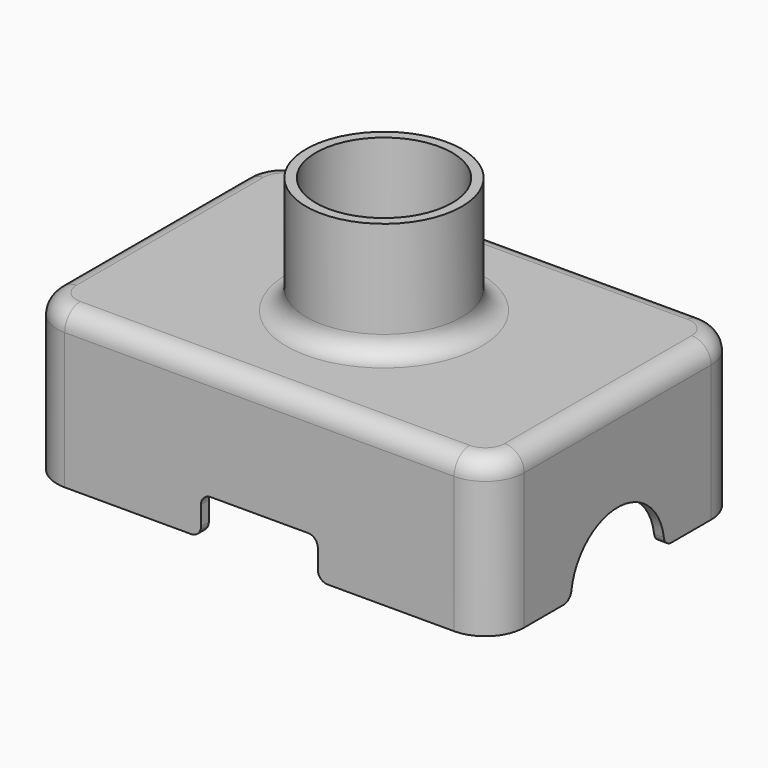
from build123d import *

# Parameters (mm, degrees)
F0_W         = 152.4
F0_H         = 101.6
F1_DEPTH     = 50.8
F2_R         = 25.4
F3_DEPTH     = 38.1
F4_R         = 12.7
F5_R         = 6.35
F6_T         = -3.175
F8_DEPTH     = 3.175
F9_W         = 38.1
F9_H         = 25.4
F10_DEPTH    = 3.175
F11_T1_DEPTH = 3.175
F11_T3_DEPTH = 17.9102262806
F11_T5_DEPTH = 19.05


# Not quite as in the source:
# - a fillet or chamfer that OpenCascade refuses, or shapes differently, is made with other operations: its cross-section is extruded or revolved along the edge and cut away or added


with BuildPart() as f1:
    # F0 (on Top) → F1 (new body)
    with BuildSketch(Plane.XY):
        Rectangle(F0_W, F0_H)
    extrude(amount=F1_DEPTH)

    # F2 (on face) → F3 (join)
    with BuildSketch(Plane.XY.offset(50.8)):
        Circle(F2_R)
    extrude(amount=F3_DEPTH)

    # F4
    f4_edges = [f1.edges().sort_by_distance(p)[0] for p in [
        (-76.2, -50.8, 25.4),
        (76.2, -50.8, 25.4),
        (76.2, 50.8, 25.4),
        (-76.2, 50.8, 25.4),
    ]]
    fillet(f4_edges, radius=F4_R)

    # F5
    f5_edges = [f1.edges().sort_by_distance(p)[0] for p in [
        (-25.4, 0, 50.8),
        (76.2, 0, 50.8),
        (72.480256, -47.080256, 50.8),
        (72.480256, 47.080256, 50.8),
        (0, -50.8, 50.8),
        (0, 50.8, 50.8),
        (-72.480256, -47.080256, 50.8),
        (-72.480256, 47.080256, 50.8),
        (-76.2, 0, 50.8),
    ]]
    fillet(f5_edges, radius=F5_R)

    # F6
    f6_openings = [f1.faces().sort_by_distance(p)[0] for p in [
        (0, 0, 0),
        (0, 0, 88.9),
    ]]
    offset(amount=F6_T, openings=f6_openings)

    # F7 (on face) → F8 (cut, through all)
    with BuildSketch(Plane.YZ.offset(76.2)):
        with BuildLine():
            Line((-19.05, 0), (19.05, 0))
            ThreePointArc((19.05, 0), (0, 19.05), (-19.05, 0))
        make_face()
    extrude(amount=-F8_DEPTH, mode=Mode.SUBTRACT)

    # F9 (on face) → F10 (cut, through all)
    with BuildSketch(Plane.XZ.offset(50.8)):
        Rectangle(F9_W, F9_H)
    extrude(amount=-F10_DEPTH, mode=Mode.SUBTRACT)

    # F11: fillet of radius 3.175 on 8 edges, made by hand

    # F11_s2 → F11_t1 (join)
    with BuildSketch(Plane.XZ.offset(47.625)):
        with BuildLine():
            ThreePointArc((-19.05, 9.525), (-18.1200640303, 11.7700640303), (-15.875, 12.7))
            Line((-15.875, 12.7), (-19.05, 12.7))
            Line((-19.05, 12.7), (-19.05, 9.525))
        make_face()
        with BuildLine():
            ThreePointArc((19.05, 9.525), (18.1200640303, 11.7700640303), (15.875, 12.7))
            Line((15.875, 12.7), (19.05, 12.7))
            Line((19.05, 12.7), (19.05, 9.525))
        make_face()
    extrude(amount=F11_T1_DEPTH)

    # F11_s4 → F11_t3 (cut)
    with BuildSketch(Plane.YZ.offset(65.6573868597)):
        with BuildLine():
            ThreePointArc((-21.9970452561, 0), (-19.9185198516, 0.7749255964), (-18.8546102195, 2.7214285714))
            ThreePointArc((-18.8546102195, 2.7214285714), (-19.0010897672, 1.3642168665), (-19.05, 0))
            Line((-19.05, 0), (-21.9970452561, 0))
        make_face()
        with BuildLine():
            ThreePointArc((18.8546102195, 2.7214285714), (19.9185198516, 0.7749255964), (21.9970452561, 0))
            Line((21.9970452561, 0), (19.05, 0))
            ThreePointArc((19.05, 0), (19.0010897672, 1.3642168665), (18.8546102195, 2.7214285714))
        make_face()
    extrude(amount=F11_T3_DEPTH, mode=Mode.SUBTRACT)

    # F11_s6 → F11_t5 (cut)
    with BuildSketch(Plane.XZ.offset(39.6875)):
        with BuildLine():
            ThreePointArc((22.225, 0), (19.9799359697, 0.9299359697), (19.05, 3.175))
            Line((19.05, 3.175), (19.05, 0))
            Line((19.05, 0), (22.225, 0))
        make_face()
        with BuildLine():
            ThreePointArc((-22.225, 0), (-19.9799359697, 0.9299359697), (-19.05, 3.175))
            Line((-19.05, 3.175), (-19.05, 0))
            Line((-19.05, 0), (-22.225, 0))
        make_face()
    extrude(amount=F11_T5_DEPTH, mode=Mode.SUBTRACT)


solid = f1.part
